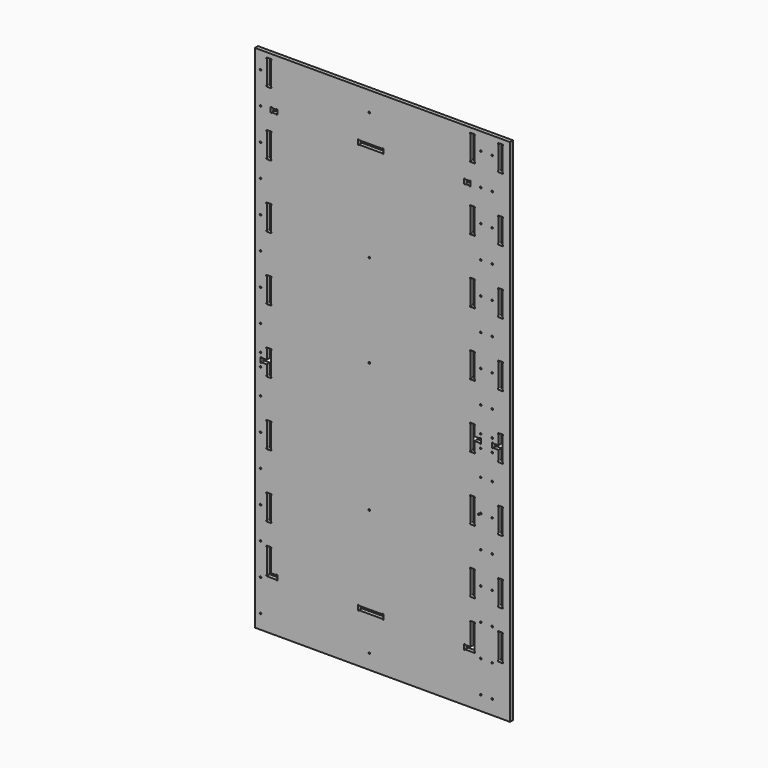
from build123d import *

# Parameters (mm, degrees)
F1_DEPTH = 18


# Not quite as in the source:
# - ends of sketch curves that miss each other by under 0.0002 mm in the source are joined


with BuildPart() as f1:
    # F0 (on Front) → F1 (new body)
    with BuildSketch(Plane.XZ):
        Polygon((-600, 1199.490696), (-600, -1200), (599.527337, -1200), (599.50121, 1199.503749), align=None)
        with BuildLine():
            ThreePointArc((-573.493655, -1128.773735), (-570.8420045706, -1129.8720845706), (-569.743655, -1132.523735))
            ThreePointArc((-569.743655, -1132.523735), (-570.8420045706, -1135.1753854294), (-573.493655, -1136.273735))
            ThreePointArc((-573.493655, -1136.273735), (-576.1453054294, -1135.1753854294), (-577.243655, -1132.523735))
            ThreePointArc((-577.243655, -1132.523735), (-576.1453054294, -1129.8720845706), (-573.493655, -1128.773735))
        make_face(mode=Mode.SUBTRACT)
        with BuildLine():
            ThreePointArc((-573.493655, -978.773735), (-570.8420045706, -979.8720845706), (-569.743655, -982.523735))
            ThreePointArc((-569.743655, -982.523735), (-570.8420045706, -985.1753854294), (-573.493655, -986.273735))
            ThreePointArc((-573.493655, -986.273735), (-576.1453054294, -985.1753854294), (-577.243655, -982.523735))
            ThreePointArc((-577.243655, -982.523735), (-576.1453054294, -979.8720845706), (-573.493655, -978.773735))
        make_face(mode=Mode.SUBTRACT)
        with BuildLine():
            ThreePointArc((-543.727655065, -848.5071848473), (-546.7362958526, -845.1312101747), (-543.477726, -841.9957920376))
            Line((-543.477726, -841.9957920376), (-524.977539, -841.99559))
            ThreePointArc((-524.977539, -841.99559), (-521.7198869029, -845.1309746571), (-524.7274680238, -848.5069766909))
            Line((-524.7274680238, -848.5069766909), (-524.726366, -949.761986))
            Line((-524.726366, -949.761986), (-500.237725, -949.76172))
            ThreePointArc((-500.237725, -949.76172), (-496.8617502129, -946.7530791459), (-493.7263320376, -950.011649))
            Line((-493.7263320376, -950.011649), (-493.726131, -968.511667))
            ThreePointArc((-493.726131, -968.511667), (-496.8615156571, -971.7693190971), (-500.2375176909, -968.7617379762))
            Line((-500.2375176909, -968.7617379762), (-543.476346, -968.762208))
            ThreePointArc((-543.476346, -968.762208), (-546.7339980971, -965.6268233429), (-543.7264169762, -962.2508213091))
            Line((-543.7264169762, -962.2508213091), (-543.727655065, -848.5071848473))
        make_face(mode=Mode.SUBTRACT)
        with BuildLine():
            ThreePointArc((-573.493655, -828.773735), (-570.8420045706, -829.8720845706), (-569.743655, -832.523735))
            ThreePointArc((-569.743655, -832.523735), (-570.8420045706, -835.1753854294), (-573.493655, -836.273735))
            ThreePointArc((-573.493655, -836.273735), (-576.1453054294, -835.1753854294), (-577.243655, -832.523735))
            ThreePointArc((-577.243655, -832.523735), (-576.1453054294, -829.8720845706), (-573.493655, -828.773735))
        make_face(mode=Mode.SUBTRACT)
        with BuildLine():
            ThreePointArc((-573.493655, -678.773735), (-570.8420045706, -679.8720845706), (-569.743655, -682.523735))
            ThreePointArc((-569.743655, -682.523735), (-570.8420045706, -685.1753854294), (-573.493655, -686.273735))
            ThreePointArc((-573.493655, -686.273735), (-576.1453054294, -685.1753854294), (-577.243655, -682.523735))
            ThreePointArc((-577.243655, -682.523735), (-576.1453054294, -679.8720845706), (-573.493655, -678.773735))
        make_face(mode=Mode.SUBTRACT)
        with BuildLine():
            ThreePointArc((-524.980091, -621.9929560323), (-521.7224389029, -625.1283406571), (-524.7300200238, -628.5043426909))
            Line((-524.7300200238, -628.5043426909), (-524.728845, -736.481683))
            ThreePointArc((-524.728845, -736.481683), (-521.7202041651, -739.8576582867), (-524.978775, -742.9930759623))
            Line((-524.978775, -742.9930759623), (-543.478594, -742.993277))
            ThreePointArc((-543.478594, -742.993277), (-546.7362460971, -739.8578923429), (-543.7286649762, -736.4818903091))
            Line((-543.7286649762, -736.4818903091), (-543.72984, -628.50455))
            ThreePointArc((-543.72984, -628.50455), (-546.7384808541, -625.1285752129), (-543.479911, -621.9931570376))
            Line((-543.479911, -621.9931570376), (-524.980091, -621.9929560323))
        make_face(mode=Mode.SUBTRACT)
        with BuildLine():
            ThreePointArc((-65.644873, -1130.966953), (-64.5465234294, -1128.3153025706), (-61.894873, -1127.216953))
            ThreePointArc((-61.894873, -1127.216953), (-59.2432225706, -1128.3153025706), (-58.144873, -1130.966953))
            ThreePointArc((-58.144873, -1130.966953), (-59.2432225706, -1133.6186034294), (-61.894873, -1134.716953))
            ThreePointArc((-61.894873, -1134.716953), (-64.5465234294, -1133.6186034294), (-65.644873, -1130.966953))
        make_face(mode=Mode.SUBTRACT)
        with BuildLine():
            ThreePointArc((-116.2255609677, -950.007539), (-113.0901763429, -946.7498869029), (-109.7141743091, -949.7574680238))
            Line((-109.7141743091, -949.7574680238), (-1.737032, -949.756293))
            ThreePointArc((-1.737032, -949.756293), (1.6389427871, -946.7476521459), (4.7743609624, -950.006222))
            Line((4.7743609624, -950.006222), (4.774562, -968.50624))
            ThreePointArc((4.774562, -968.50624), (1.6391773429, -971.7638920971), (-1.7368246909, -968.7563109762))
            Line((-1.7368246909, -968.7563109762), (-109.713967, -968.757486))
            ThreePointArc((-109.713967, -968.757486), (-113.0899408253, -971.7661268526), (-116.2253589624, -968.507557))
            Line((-116.2253589624, -968.507557), (-116.2255609677, -950.007539))
        make_face(mode=Mode.SUBTRACT)
        with BuildLine():
            ThreePointArc((-573.493655, -528.773735), (-570.8420045706, -529.8720845706), (-569.743655, -532.523735))
            ThreePointArc((-569.743655, -532.523735), (-570.8420045706, -535.1753854294), (-573.493655, -536.273735))
            ThreePointArc((-573.493655, -536.273735), (-576.1453054294, -535.1753854294), (-577.243655, -532.523735))
            ThreePointArc((-577.243655, -532.523735), (-576.1453054294, -529.8720845706), (-573.493655, -528.773735))
        make_face(mode=Mode.SUBTRACT)
        with BuildLine():
            ThreePointArc((-573.493655, -378.773735), (-570.8420045706, -379.8720845706), (-569.743655, -382.523735))
            ThreePointArc((-569.743655, -382.523735), (-570.8420045706, -385.1753854294), (-573.493655, -386.273735))
            ThreePointArc((-573.493655, -386.273735), (-576.1453054294, -385.1753854294), (-577.243655, -382.523735))
            ThreePointArc((-577.243655, -382.523735), (-576.1453054294, -379.8720845706), (-573.493655, -378.773735))
        make_face(mode=Mode.SUBTRACT)
        with BuildLine():
            ThreePointArc((-524.983356, -321.9926560323), (-521.7257039029, -325.1280406571), (-524.7332850238, -328.5040426909))
            Line((-524.7332850238, -328.5040426909), (-524.73211, -436.481383))
            ThreePointArc((-524.73211, -436.481383), (-521.7234691459, -439.8573577871), (-524.982039, -442.9927759624))
            Line((-524.982039, -442.9927759624), (-543.481858, -442.992977))
            ThreePointArc((-543.481858, -442.992977), (-546.7395100971, -439.8575923429), (-543.7319289762, -436.4815903091))
            Line((-543.7319289762, -436.4815903091), (-543.733104, -328.50425))
            ThreePointArc((-543.733104, -328.50425), (-546.7417448541, -325.1282752129), (-543.483175, -321.9928570376))
            Line((-543.483175, -321.9928570376), (-524.983356, -321.9926560323))
        make_face(mode=Mode.SUBTRACT)
        with BuildLine():
            ThreePointArc((-573.493655, -228.773735), (-570.8420045706, -229.8720845706), (-569.743655, -232.523735))
            ThreePointArc((-569.743655, -232.523735), (-570.8420045706, -235.1753854294), (-573.493655, -236.273735))
            ThreePointArc((-573.493655, -236.273735), (-576.1453054294, -235.1753854294), (-577.243655, -232.523735))
            ThreePointArc((-577.243655, -232.523735), (-576.1453054294, -229.8720845706), (-573.493655, -228.773735))
        make_face(mode=Mode.SUBTRACT)
        with BuildLine():
            ThreePointArc((-573.493655, -108.773735), (-570.8420045706, -109.8720845706), (-569.743655, -112.523735))
            ThreePointArc((-569.743655, -112.523735), (-570.8420045706, -115.1753854294), (-573.493655, -116.273735))
            ThreePointArc((-573.493655, -116.273735), (-576.1453054294, -115.1753854294), (-577.243655, -112.523735))
            ThreePointArc((-577.243655, -112.523735), (-576.1453054294, -109.8720845706), (-573.493655, -108.773735))
        make_face(mode=Mode.SUBTRACT)
        with BuildLine():
            ThreePointArc((-524.98662, -21.9923560324), (-521.7289688837, -25.1277411567), (-524.7365500238, -28.5037426909))
            Line((-524.7365500238, -28.5037426909), (-524.735375, -136.481083))
            ThreePointArc((-524.735375, -136.481083), (-521.7267341459, -139.8570577871), (-524.985304, -142.9924759624))
            Line((-524.985304, -142.9924759624), (-543.485097, -142.992677))
            ThreePointArc((-543.485097, -142.992677), (-546.7429566344, -139.8575125023), (-543.7356079554, -136.4813075779))
            Line((-543.7356079554, -136.4813075779), (-543.73916, -91.996839))
            Line((-543.73916, -91.996839), (-568.227835, -91.997105))
            ThreePointArc((-568.227835, -91.997105), (-571.6038097871, -95.0057458541), (-574.7392279624, -91.747176))
            Line((-574.7392279624, -91.747176), (-574.739429, -73.247158))
            ThreePointArc((-574.739429, -73.247158), (-571.6040443429, -69.9895059029), (-568.2280423091, -72.9970870238))
            Line((-568.2280423091, -72.9970870238), (-543.739563, -72.996821))
            Line((-543.739563, -72.996821), (-543.736807, -28.503931))
            ThreePointArc((-543.736807, -28.503931), (-546.7452018944, -25.1277420055), (-543.486412, -21.9925570804))
            Line((-543.486412, -21.9925570804), (-524.98662, -21.9923560324))
        make_face(mode=Mode.SUBTRACT)
        with BuildLine():
            ThreePointArc((-573.493655, -48.773735), (-570.8420045706, -49.8720845706), (-569.743655, -52.523735))
            ThreePointArc((-569.743655, -52.523735), (-570.8420045706, -55.1753854294), (-573.493655, -56.273735))
            ThreePointArc((-573.493655, -56.273735), (-576.1453054294, -55.1753854294), (-577.243655, -52.523735))
            ThreePointArc((-577.243655, -52.523735), (-576.1453054294, -49.8720845706), (-573.493655, -48.773735))
        make_face(mode=Mode.SUBTRACT)
        with BuildLine():
            ThreePointArc((-65.644873, -537.813487), (-64.5465234294, -535.1618365706), (-61.894873, -534.063487))
            ThreePointArc((-61.894873, -534.063487), (-59.2432225706, -535.1618365706), (-58.144873, -537.813487))
            ThreePointArc((-58.144873, -537.813487), (-59.2432225706, -540.4651374294), (-61.894873, -541.563487))
            ThreePointArc((-61.894873, -541.563487), (-64.5465234294, -540.4651374294), (-65.644873, -537.813487))
        make_face(mode=Mode.SUBTRACT)
        with BuildLine():
            ThreePointArc((413.2732930585, -848.4955412375), (410.2646479537, -845.1195722402), (413.523212, -841.9841500368))
            Line((413.523212, -841.9841500368), (432.023061, -841.983948))
            ThreePointArc((432.023061, -841.983948), (435.2807130971, -845.1193326571), (432.2731319762, -848.4953346909))
            Line((432.2731319762, -848.4953346909), (432.27437, -962.240198))
            ThreePointArc((432.27437, -962.240198), (435.2830108541, -965.6161727871), (432.024441, -968.7515909624))
            Line((432.024441, -968.7515909624), (388.786108, -968.752061))
            ThreePointArc((388.786108, -968.752061), (385.4101332129, -971.7607018541), (382.2747150376, -968.502132))
            Line((382.2747150376, -968.502132), (382.274514, -950.002325))
            ThreePointArc((382.274514, -950.002325), (385.4098986571, -946.7446729029), (388.7859006909, -949.7522540238))
            Line((388.7859006909, -949.7522540238), (413.274542, -949.751987))
            Line((413.274542, -949.751987), (413.2732930585, -848.4955412375))
        make_face(mode=Mode.SUBTRACT)
        with BuildLine():
            ThreePointArc((461.992992, -1128.773735), (464.6446424294, -1129.8720845706), (465.742992, -1132.523735))
            ThreePointArc((465.742992, -1132.523735), (464.6446424294, -1135.1753854294), (461.992992, -1136.273735))
            ThreePointArc((461.992992, -1136.273735), (459.3413415706, -1135.1753854294), (458.242992, -1132.523735))
            ThreePointArc((458.242992, -1132.523735), (459.3413415706, -1129.8720845706), (461.992992, -1128.773735))
        make_face(mode=Mode.SUBTRACT)
        with BuildLine():
            ThreePointArc((515.501657, -1128.773735), (518.1533074294, -1129.8720845706), (519.251657, -1132.523735))
            ThreePointArc((519.251657, -1132.523735), (518.1533074294, -1135.1753854294), (515.501657, -1136.273735))
            ThreePointArc((515.501657, -1136.273735), (512.8500065706, -1135.1753854294), (511.751657, -1132.523735))
            ThreePointArc((511.751657, -1132.523735), (512.8500065706, -1129.8720845706), (515.501657, -1128.773735))
        make_face(mode=Mode.SUBTRACT)
        with BuildLine():
            ThreePointArc((461.992992, -978.773735), (464.6446424294, -979.8720845706), (465.742992, -982.523735))
            ThreePointArc((465.742992, -982.523735), (464.6446424294, -985.1753854294), (461.992992, -986.273735))
            ThreePointArc((461.992992, -986.273735), (459.3413415706, -985.1753854294), (458.242992, -982.523735))
            ThreePointArc((458.242992, -982.523735), (459.3413415706, -979.8720845706), (461.992992, -978.773735))
        make_face(mode=Mode.SUBTRACT)
        with BuildLine():
            ThreePointArc((515.501657, -978.773735), (518.1533074294, -979.8720845706), (519.251657, -982.523735))
            ThreePointArc((519.251657, -982.523735), (518.1533074294, -985.1753854294), (515.501657, -986.273735))
            ThreePointArc((515.501657, -986.273735), (512.8500065706, -985.1753854294), (511.751657, -982.523735))
            ThreePointArc((511.751657, -982.523735), (512.8500065706, -979.8720845706), (515.501657, -978.773735))
        make_face(mode=Mode.SUBTRACT)
        with BuildLine():
            Line((545.274457, -962.243698), (545.273219, -848.49533))
            ThreePointArc((545.273219, -848.49533), (542.2645781474, -845.1193561747), (545.523148, -841.9839380376))
            Line((545.523148, -841.9839380376), (564.022958, -841.983736))
            ThreePointArc((564.022958, -841.983736), (567.2806100971, -845.1191206571), (564.2730289762, -848.4951226909))
            Line((564.2730289762, -848.4951226909), (564.274266, -962.243491))
            ThreePointArc((564.274266, -962.243491), (567.2829068541, -965.6194657871), (564.024337, -968.7548839624))
            Line((564.024337, -968.7548839624), (545.524528, -968.755085))
            ThreePointArc((545.524528, -968.755085), (542.2668759029, -965.6197003429), (545.274457, -962.243698))
        make_face(mode=Mode.SUBTRACT)
        with BuildLine():
            ThreePointArc((413.522136, -742.9794189677), (410.2644839029, -739.8440343429), (413.2720650238, -736.4680323091))
            Line((413.2720650238, -736.4680323091), (413.27089, -628.49064))
            ThreePointArc((413.27089, -628.49064), (410.2622491459, -625.1146652129), (413.520819, -621.9792470376))
            Line((413.520819, -621.9792470376), (432.020837, -621.979046))
            ThreePointArc((432.020837, -621.979046), (435.2784890971, -625.1144306571), (432.2709079762, -628.4904326909))
            Line((432.2709079762, -628.4904326909), (432.272083, -736.467825))
            ThreePointArc((432.272083, -736.467825), (435.2807238526, -739.8437988253), (432.022154, -742.9792169624))
            Line((432.022154, -742.9792169624), (413.522136, -742.9794189677))
        make_face(mode=Mode.SUBTRACT)
        with BuildLine():
            ThreePointArc((461.992992, -828.773735), (464.6446424294, -829.8720845706), (465.742992, -832.523735))
            ThreePointArc((465.742992, -832.523735), (464.6446424294, -835.1753854294), (461.992992, -836.273735))
            ThreePointArc((461.992992, -836.273735), (459.3413415706, -835.1753854294), (458.242992, -832.523735))
            ThreePointArc((458.242992, -832.523735), (459.3413415706, -829.8720845706), (461.992992, -828.773735))
        make_face(mode=Mode.SUBTRACT)
        with BuildLine():
            ThreePointArc((515.501657, -828.773735), (518.1533074294, -829.8720845706), (519.251657, -832.523735))
            ThreePointArc((519.251657, -832.523735), (518.1533074294, -835.1753854294), (515.501657, -836.273735))
            ThreePointArc((515.501657, -836.273735), (512.8500065706, -835.1753854294), (511.751657, -832.523735))
            ThreePointArc((511.751657, -832.523735), (512.8500065706, -829.8720845706), (515.501657, -828.773735))
        make_face(mode=Mode.SUBTRACT)
        with BuildLine():
            ThreePointArc((461.992992, -678.773735), (464.6446424294, -679.8720845706), (465.742992, -682.523735))
            ThreePointArc((465.742992, -682.523735), (464.6446424294, -685.1753854294), (461.992992, -686.273735))
            ThreePointArc((461.992992, -686.273735), (459.3413415706, -685.1753854294), (458.242992, -682.523735))
            ThreePointArc((458.242992, -682.523735), (459.3413415706, -679.8720845706), (461.992992, -678.773735))
        make_face(mode=Mode.SUBTRACT)
        with BuildLine():
            ThreePointArc((515.501657, -678.773735), (518.1533074294, -679.8720845706), (519.251657, -682.523735))
            ThreePointArc((519.251657, -682.523735), (518.1533074294, -685.1753854294), (515.501657, -686.273735))
            ThreePointArc((515.501657, -686.273735), (512.8500065706, -685.1753854294), (511.751657, -682.523735))
            ThreePointArc((511.751657, -682.523735), (512.8500065706, -679.8720845706), (515.501657, -678.773735))
        make_face(mode=Mode.SUBTRACT)
        with BuildLine():
            ThreePointArc((545.522316, -742.9779789677), (542.2646629037, -739.8425933813), (545.272244947, -736.4665903121))
            Line((545.272244947, -736.4665903121), (545.27107, -628.489199))
            ThreePointArc((545.27107, -628.489199), (542.2624291459, -625.1132242129), (545.520999, -621.9778060376))
            Line((545.520999, -621.9778060376), (564.020799, -621.977605))
            ThreePointArc((564.020799, -621.977605), (567.2784510971, -625.1129896571), (564.2708699762, -628.4889916909))
            Line((564.2708699762, -628.4889916909), (564.272045, -736.466332))
            ThreePointArc((564.272045, -736.466332), (567.2806858526, -739.8423058253), (564.022116, -742.9777239624))
            Line((564.022116, -742.9777239624), (545.522316, -742.9779789677))
        make_face(mode=Mode.SUBTRACT)
        with BuildLine():
            ThreePointArc((432.268818065, -436.4675241527), (435.2774588526, -439.8434988253), (432.018889, -442.9789169624))
            Line((432.018889, -442.9789169624), (413.518871, -442.979119))
            ThreePointArc((413.518871, -442.979119), (410.2612189029, -439.8437343429), (413.2688000238, -436.4677323091))
            Line((413.2688000238, -436.4677323091), (413.267625, -328.49034))
            ThreePointArc((413.267625, -328.49034), (410.2589841459, -325.1143652129), (413.517554, -321.9789470376))
            Line((413.517554, -321.9789470376), (432.017572, -321.978746))
            ThreePointArc((432.017572, -321.978746), (435.2752240971, -325.1141306571), (432.2676429762, -328.4901326909))
            Line((432.2676429762, -328.4901326909), (432.268818065, -436.4675241527))
        make_face(mode=Mode.SUBTRACT)
        with BuildLine():
            ThreePointArc((461.992992, -528.773735), (464.6446424294, -529.8720845706), (465.742992, -532.523735))
            ThreePointArc((465.742992, -532.523735), (464.6446424294, -535.1753854294), (461.992992, -536.273735))
            ThreePointArc((461.992992, -536.273735), (459.3413415706, -535.1753854294), (458.242992, -532.523735))
            ThreePointArc((458.242992, -532.523735), (459.3413415706, -529.8720845706), (461.992992, -528.773735))
        make_face(mode=Mode.SUBTRACT)
        with BuildLine():
            ThreePointArc((515.501657, -528.773735), (518.1533074294, -529.8720845706), (519.251657, -532.523735))
            ThreePointArc((519.251657, -532.523735), (518.1533074294, -535.1753854294), (515.501657, -536.273735))
            ThreePointArc((515.501657, -536.273735), (512.8500065706, -535.1753854294), (511.751657, -532.523735))
            ThreePointArc((511.751657, -532.523735), (512.8500065706, -529.8720845706), (515.501657, -528.773735))
        make_face(mode=Mode.SUBTRACT)
        with BuildLine():
            ThreePointArc((447.984, -388.548053), (449.0823495706, -385.8964025706), (451.734, -384.798053))
            ThreePointArc((451.734, -384.798053), (454.3856504294, -385.8964025706), (455.484, -388.548053))
            ThreePointArc((455.484, -388.548053), (454.3856504294, -391.1997034294), (451.734, -392.298053))
            ThreePointArc((451.734, -392.298053), (449.0823495706, -391.1997034294), (447.984, -388.548053))
        make_face(mode=Mode.SUBTRACT)
        with BuildLine():
            ThreePointArc((461.992992, -378.773735), (464.6446424294, -379.8720845706), (465.742992, -382.523735))
            ThreePointArc((465.742992, -382.523735), (464.6446424294, -385.1753854294), (461.992992, -386.273735))
            ThreePointArc((461.992992, -386.273735), (459.3413415706, -385.1753854294), (458.242992, -382.523735))
            ThreePointArc((458.242992, -382.523735), (459.3413415706, -379.8720845706), (461.992992, -378.773735))
        make_face(mode=Mode.SUBTRACT)
        with BuildLine():
            ThreePointArc((515.501657, -378.773735), (518.1533074294, -379.8720845706), (519.251657, -382.523735))
            ThreePointArc((519.251657, -382.523735), (518.1533074294, -385.1753854294), (515.501657, -386.273735))
            ThreePointArc((515.501657, -386.273735), (512.8500065706, -385.1753854294), (511.751657, -382.523735))
            ThreePointArc((511.751657, -382.523735), (512.8500065706, -379.8720845706), (515.501657, -378.773735))
        make_face(mode=Mode.SUBTRACT)
        with BuildLine():
            ThreePointArc((545.519052, -442.9776789677), (542.2613989228, -439.8422938795), (545.2689799529, -436.4662903887))
            Line((545.2689799529, -436.4662903887), (545.267805, -328.488899))
            ThreePointArc((545.267805, -328.488899), (542.2591641651, -325.1129237133), (545.517735, -321.9775060377))
            Line((545.517735, -321.9775060377), (564.017534, -321.977305))
            ThreePointArc((564.017534, -321.977305), (567.2751860971, -325.1126896571), (564.2676049762, -328.4886916909))
            Line((564.2676049762, -328.4886916909), (564.26878, -436.466032))
            ThreePointArc((564.26878, -436.466032), (567.2774208526, -439.8420058253), (564.018851, -442.9774239624))
            Line((564.018851, -442.9774239624), (545.519052, -442.9776789677))
        make_face(mode=Mode.SUBTRACT)
        with BuildLine():
            ThreePointArc((432.2652829744, -136.4718953334), (435.2740837852, -139.8477271674), (432.015663, -142.9832999823))
            Line((432.015663, -142.9832999823), (413.515627, -142.983501))
            ThreePointArc((413.515627, -142.983501), (410.2579749029, -139.8481163429), (413.2655560238, -136.4721143091))
            Line((413.2655560238, -136.4721143091), (413.264381, -28.494722))
            ThreePointArc((413.264381, -28.494722), (410.2557401666, -25.1187476751), (413.514311, -21.9833300377))
            Line((413.514311, -21.9833300377), (432.014348, -21.983128))
            ThreePointArc((432.014348, -21.983128), (435.2718385306, -25.1186802863), (432.2640839659, -28.4945275573))
            Line((432.2640839659, -28.4945275573), (432.262235, -72.9862))
            Line((432.262235, -72.9862), (456.75085, -72.985934))
            ThreePointArc((456.75085, -72.985934), (460.1268238253, -69.9772931474), (463.2622419624, -73.235863))
            Line((463.2622419624, -73.235863), (463.262444, -91.735881))
            ThreePointArc((463.262444, -91.735881), (460.1270593429, -94.9935330971), (456.7510573091, -91.9859519762))
            Line((456.7510573091, -91.9859519762), (432.262638, -91.986218))
            Line((432.262638, -91.986218), (432.2652829744, -136.4718953334))
        make_face(mode=Mode.SUBTRACT)
        with BuildLine():
            ThreePointArc((461.992992, -228.773735), (464.6446424294, -229.8720845706), (465.742992, -232.523735))
            ThreePointArc((465.742992, -232.523735), (464.6446424294, -235.1753854294), (461.992992, -236.273735))
            ThreePointArc((461.992992, -236.273735), (459.3413415706, -235.1753854294), (458.242992, -232.523735))
            ThreePointArc((458.242992, -232.523735), (459.3413415706, -229.8720845706), (461.992992, -228.773735))
        make_face(mode=Mode.SUBTRACT)
        with BuildLine():
            ThreePointArc((515.501657, -228.773735), (518.1533074294, -229.8720845706), (519.251657, -232.523735))
            ThreePointArc((519.251657, -232.523735), (518.1533074294, -235.1753854294), (515.501657, -236.273735))
            ThreePointArc((515.501657, -236.273735), (512.8500065706, -235.1753854294), (511.751657, -232.523735))
            ThreePointArc((511.751657, -232.523735), (512.8500065706, -229.8720845706), (515.501657, -228.773735))
        make_face(mode=Mode.SUBTRACT)
        with BuildLine():
            ThreePointArc((461.992992, -108.773735), (464.6446424294, -109.8720845706), (465.742992, -112.523735))
            ThreePointArc((465.742992, -112.523735), (464.6446424294, -115.1753854294), (461.992992, -116.273735))
            ThreePointArc((461.992992, -116.273735), (459.3413415706, -115.1753854294), (458.242992, -112.523735))
            ThreePointArc((458.242992, -112.523735), (459.3413415706, -109.8720845706), (461.992992, -108.773735))
        make_face(mode=Mode.SUBTRACT)
        with BuildLine():
            ThreePointArc((515.501657, -108.773735), (518.1533074294, -109.8720845706), (519.251657, -112.523735))
            ThreePointArc((519.251657, -112.523735), (518.1533074294, -115.1753854294), (515.501657, -116.273735))
            ThreePointArc((515.501657, -116.273735), (512.8500065706, -115.1753854294), (511.751657, -112.523735))
            ThreePointArc((511.751657, -112.523735), (512.8500065706, -109.8720845706), (515.501657, -108.773735))
        make_face(mode=Mode.SUBTRACT)
        with BuildLine():
            ThreePointArc((461.992992, -48.773735), (464.6446424294, -49.8720845706), (465.742992, -52.523735))
            ThreePointArc((465.742992, -52.523735), (464.6446424294, -55.1753854294), (461.992992, -56.273735))
            ThreePointArc((461.992992, -56.273735), (459.3413415706, -55.1753854294), (458.242992, -52.523735))
            ThreePointArc((458.242992, -52.523735), (459.3413415706, -49.8720845706), (461.992992, -48.773735))
        make_face(mode=Mode.SUBTRACT)
        with BuildLine():
            ThreePointArc((515.501657, -48.773735), (518.1533074294, -49.8720845706), (519.251657, -52.523735))
            ThreePointArc((519.251657, -52.523735), (518.1533074294, -55.1753854294), (515.501657, -56.273735))
            ThreePointArc((515.501657, -56.273735), (512.8500065706, -55.1753854294), (511.751657, -52.523735))
            ThreePointArc((511.751657, -52.523735), (512.8500065706, -49.8720845706), (515.501657, -48.773735))
        make_face(mode=Mode.SUBTRACT)
        with BuildLine():
            ThreePointArc((545.513838, -142.9839189899), (542.2559918459, -139.8487409931), (545.2633540444, -136.4725485752))
            Line((545.2633540444, -136.4725485752), (545.25999, -91.98499))
            Line((545.25999, -91.98499), (520.771316, -91.985256))
            ThreePointArc((520.771316, -91.985256), (517.3953421747, -94.9938968526), (514.2599240376, -91.735327))
            Line((514.2599240376, -91.735327), (514.259723, -73.235309))
            ThreePointArc((514.259723, -73.235309), (517.3951076571, -69.9776569029), (520.7711096909, -72.9852380238))
            Line((520.7711096909, -72.9852380238), (545.259783, -72.984972))
            Line((545.259783, -72.984972), (545.262179, -28.495176))
            ThreePointArc((545.262179, -28.495176), (542.2537571036, -25.1190100629), (545.512522, -21.9837990747))
            Line((545.512522, -21.9837990747), (564.012515, -21.983598))
            ThreePointArc((564.012515, -21.983598), (567.2701670971, -25.1189826571), (564.2625859762, -28.4949846909))
            Line((564.2625859762, -28.4949846909), (564.263761, -136.472325))
            ThreePointArc((564.263761, -136.472325), (567.2724018541, -139.8482997871), (564.013832, -142.9837179624))
            Line((564.013832, -142.9837179624), (545.513838, -142.9839189899))
        make_face(mode=Mode.SUBTRACT)
        with BuildLine():
            ThreePointArc((-573.493655, 71.226265), (-570.8420045706, 70.1279154294), (-569.743655, 67.476265))
            ThreePointArc((-569.743655, 67.476265), (-570.8420045706, 64.8246145706), (-573.493655, 63.726265))
            ThreePointArc((-573.493655, 63.726265), (-576.1453054294, 64.8246145706), (-577.243655, 67.476265))
            ThreePointArc((-577.243655, 67.476265), (-576.1453054294, 70.1279154294), (-573.493655, 71.226265))
        make_face(mode=Mode.SUBTRACT)
        with BuildLine():
            ThreePointArc((-573.493655, 221.226265), (-570.8420045706, 220.1279154294), (-569.743655, 217.476265))
            ThreePointArc((-569.743655, 217.476265), (-570.8420045706, 214.8246145706), (-573.493655, 213.726265))
            ThreePointArc((-573.493655, 213.726265), (-576.1453054294, 214.8246145706), (-577.243655, 217.476265))
            ThreePointArc((-577.243655, 217.476265), (-576.1453054294, 220.1279154294), (-573.493655, 221.226265))
        make_face(mode=Mode.SUBTRACT)
        with BuildLine():
            ThreePointArc((-543.7396339887, 271.4963501468), (-546.7482748349, 274.8723252867), (-543.489704, 278.0077429623))
            Line((-543.489704, 278.0077429623), (-524.989885, 278.007944))
            ThreePointArc((-524.989885, 278.007944), (-521.7322329029, 274.8725593429), (-524.7398140238, 271.4965573091))
            Line((-524.7398140238, 271.4965573091), (-524.738639, 163.519217))
            ThreePointArc((-524.738639, 163.519217), (-521.7299981459, 160.1432422129), (-524.988568, 157.0078240376))
            Line((-524.988568, 157.0078240376), (-543.488388, 157.007623))
            ThreePointArc((-543.488388, 157.007623), (-546.7460400971, 160.1430076571), (-543.7384589762, 163.5190096909))
            Line((-543.7384589762, 163.5190096909), (-543.7396339887, 271.4963501468))
        make_face(mode=Mode.SUBTRACT)
        with BuildLine():
            ThreePointArc((-573.493655, 371.226265), (-570.8420045706, 370.1279154294), (-569.743655, 367.476265))
            ThreePointArc((-569.743655, 367.476265), (-570.8420045706, 364.8246145706), (-573.493655, 363.726265))
            ThreePointArc((-573.493655, 363.726265), (-576.1453054294, 364.8246145706), (-577.243655, 367.476265))
            ThreePointArc((-577.243655, 367.476265), (-576.1453054294, 370.1279154294), (-573.493655, 371.226265))
        make_face(mode=Mode.SUBTRACT)
        with BuildLine():
            ThreePointArc((-573.493655, 521.226265), (-570.8420045706, 520.1279154294), (-569.743655, 517.476265))
            ThreePointArc((-569.743655, 517.476265), (-570.8420045706, 514.8246145706), (-573.493655, 513.726265))
            ThreePointArc((-573.493655, 513.726265), (-576.1453054294, 514.8246145706), (-577.243655, 517.476265))
            ThreePointArc((-577.243655, 517.476265), (-576.1453054294, 520.1279154294), (-573.493655, 521.226265))
        make_face(mode=Mode.SUBTRACT)
        with BuildLine():
            ThreePointArc((-524.99315, 578.0082439677), (-521.7354979029, 574.8728593429), (-524.7430790238, 571.4968573091))
            Line((-524.7430790238, 571.4968573091), (-524.741904, 463.519517))
            ThreePointArc((-524.741904, 463.519517), (-521.7332631459, 460.1435422129), (-524.991833, 457.0081240376))
            Line((-524.991833, 457.0081240376), (-543.491652, 457.007923))
            ThreePointArc((-543.491652, 457.007923), (-546.7493040971, 460.1433076571), (-543.7417229762, 463.5193096909))
            Line((-543.7417229762, 463.5193096909), (-543.742898, 571.49665))
            ThreePointArc((-543.742898, 571.49665), (-546.7515388541, 574.8726247871), (-543.492969, 578.0080429624))
            Line((-543.492969, 578.0080429624), (-524.99315, 578.0082439677))
        make_face(mode=Mode.SUBTRACT)
        with BuildLine():
            ThreePointArc((-65.644873, 70.75488), (-64.5465234294, 73.4065304294), (-61.894873, 74.50488))
            ThreePointArc((-61.894873, 74.50488), (-59.2432225706, 73.4065304294), (-58.144873, 70.75488))
            ThreePointArc((-58.144873, 70.75488), (-59.2432225706, 68.1032295706), (-61.894873, 67.00488))
            ThreePointArc((-61.894873, 67.00488), (-64.5465234294, 68.1032295706), (-65.644873, 70.75488))
        make_face(mode=Mode.SUBTRACT)
        with BuildLine():
            ThreePointArc((-65.644873, 506.390807), (-64.5465234294, 509.0424574294), (-61.894873, 510.140807))
            ThreePointArc((-61.894873, 510.140807), (-59.2432225706, 509.0424574294), (-58.144873, 506.390807))
            ThreePointArc((-58.144873, 506.390807), (-59.2432225706, 503.7391565706), (-61.894873, 502.640807))
            ThreePointArc((-61.894873, 502.640807), (-64.5465234294, 503.7391565706), (-65.644873, 506.390807))
        make_face(mode=Mode.SUBTRACT)
        with BuildLine():
            ThreePointArc((-573.493655, 671.226265), (-570.8420045706, 670.1279154294), (-569.743655, 667.476265))
            ThreePointArc((-569.743655, 667.476265), (-570.8420045706, 664.8246145706), (-573.493655, 663.726265))
            ThreePointArc((-573.493655, 663.726265), (-576.1453054294, 664.8246145706), (-577.243655, 667.476265))
            ThreePointArc((-577.243655, 667.476265), (-576.1453054294, 670.1279154294), (-573.493655, 671.226265))
        make_face(mode=Mode.SUBTRACT)
        with BuildLine():
            ThreePointArc((-573.493655, 821.226265), (-570.8420045706, 820.1279154294), (-569.743655, 817.476265))
            ThreePointArc((-569.743655, 817.476265), (-570.8420045706, 814.8246145706), (-573.493655, 813.726265))
            ThreePointArc((-573.493655, 813.726265), (-576.1453054294, 814.8246145706), (-577.243655, 817.476265))
            ThreePointArc((-577.243655, 817.476265), (-576.1453054294, 820.1279154294), (-573.493655, 821.226265))
        make_face(mode=Mode.SUBTRACT)
        with BuildLine():
            ThreePointArc((-543.7461629887, 871.4969501468), (-546.7548038541, 874.8729247871), (-543.496234, 878.0083429624))
            Line((-543.496234, 878.0083429624), (-524.996414, 878.008544))
            ThreePointArc((-524.996414, 878.008544), (-521.7387619029, 874.8731593429), (-524.7463430238, 871.4971573091))
            Line((-524.7463430238, 871.4971573091), (-524.745168, 763.519817))
            ThreePointArc((-524.745168, 763.519817), (-521.7365271459, 760.1438422129), (-524.995097, 757.0084240376))
            Line((-524.995097, 757.0084240376), (-543.494917, 757.008223))
            ThreePointArc((-543.494917, 757.008223), (-546.7525690971, 760.1436076571), (-543.7449879762, 763.5196096909))
            Line((-543.7449879762, 763.5196096909), (-543.7461629887, 871.4969501468))
        make_face(mode=Mode.SUBTRACT)
        with BuildLine():
            ThreePointArc((-573.493655, 971.226265), (-570.8420045706, 970.1279154294), (-569.743655, 967.476265))
            ThreePointArc((-569.743655, 967.476265), (-570.8420045706, 964.8246145706), (-573.493655, 963.726265))
            ThreePointArc((-573.493655, 963.726265), (-576.1453054294, 964.8246145706), (-577.243655, 967.476265))
            ThreePointArc((-577.243655, 967.476265), (-576.1453054294, 970.1279154294), (-573.493655, 971.226265))
        make_face(mode=Mode.SUBTRACT)
        with BuildLine():
            ThreePointArc((-501.2587058532, 977.0089919887), (-497.8827312129, 980.0176328541), (-494.7473130376, 976.759063))
            Line((-494.7473130376, 976.759063), (-494.747099, 958.258901))
            ThreePointArc((-494.747099, 958.258901), (-497.8824836571, 955.0012489029), (-501.2584856909, 958.0088300238))
            Line((-501.2584856909, 958.0088300238), (-519.235546, 958.008635))
            ThreePointArc((-519.235546, 958.008635), (-522.6115193257, 954.9999941282), (-525.7469379626, 958.258563))
            Line((-525.7469379626, 958.258563), (-525.747346, 976.758724))
            ThreePointArc((-525.747346, 976.758724), (-522.6119618411, 980.016376078), (-519.2359593857, 977.0087959703))
            Line((-519.2359593857, 977.0087959703), (-501.2587058532, 977.0089919887))
        make_face(mode=Mode.SUBTRACT)
        with BuildLine():
            ThreePointArc((-573.493655, 1121.226265), (-570.8420045706, 1120.1279154294), (-569.743655, 1117.476265))
            ThreePointArc((-569.743655, 1117.476265), (-570.8420045706, 1114.8246145706), (-573.493655, 1113.726265))
            ThreePointArc((-573.493655, 1113.726265), (-576.1453054294, 1114.8246145706), (-577.243655, 1117.476265))
            ThreePointArc((-577.243655, 1117.476265), (-576.1453054294, 1120.1279154294), (-573.493655, 1121.226265))
        make_face(mode=Mode.SUBTRACT)
        with BuildLine():
            ThreePointArc((-524.7484460113, 1063.5201168532), (-521.7398051459, 1060.1441422129), (-524.998375, 1057.0087240376))
            Line((-524.998375, 1057.0087240376), (-543.498393, 1057.008523))
            ThreePointArc((-543.498393, 1057.008523), (-546.7560450971, 1060.1439076571), (-543.7484639762, 1063.5199096909))
            Line((-543.7484639762, 1063.5199096909), (-543.749639, 1171.49725))
            ThreePointArc((-543.749639, 1171.49725), (-546.7582798541, 1174.8732247871), (-543.49971, 1178.0086429624))
            Line((-543.49971, 1178.0086429624), (-524.999692, 1178.008844))
            ThreePointArc((-524.999692, 1178.008844), (-521.7420399029, 1174.8734593429), (-524.7496210238, 1171.4974573091))
            Line((-524.7496210238, 1171.4974573091), (-524.7484460113, 1063.5201168532))
        make_face(mode=Mode.SUBTRACT)
        with BuildLine():
            ThreePointArc((-1.7581598473, 977.014427065), (1.6178143257, 980.0230678718), (4.7532329626, 976.764499))
            Line((4.7532329626, 976.764499), (4.753631, 958.264321))
            ThreePointArc((4.753631, 958.264321), (1.6182468411, 955.006668922), (-1.7577556143, 958.0142490297))
            Line((-1.7577556143, 958.0142490297), (-109.734896, 958.013074))
            ThreePointArc((-109.734896, 958.013074), (-113.1108697878, 955.0044331076), (-116.2462889627, 958.263001))
            Line((-116.2462889627, 958.263001), (-116.24689, 976.763179))
            ThreePointArc((-116.24689, 976.763179), (-113.1115063407, 980.0208320588), (-109.7355033857, 977.0132519703))
            Line((-109.7355033857, 977.0132519703), (-1.7581598473, 977.014427065))
        make_face(mode=Mode.SUBTRACT)
        with BuildLine():
            ThreePointArc((-65.644873, 1107.267947), (-64.5465234294, 1109.9195974294), (-61.894873, 1111.017947))
            ThreePointArc((-61.894873, 1111.017947), (-59.2432225706, 1109.9195974294), (-58.144873, 1107.267947))
            ThreePointArc((-58.144873, 1107.267947), (-59.2432225706, 1104.6162965706), (-61.894873, 1103.517947))
            ThreePointArc((-61.894873, 1103.517947), (-64.5465234294, 1104.6162965706), (-65.644873, 1107.267947))
        make_face(mode=Mode.SUBTRACT)
        with BuildLine():
            ThreePointArc((432.262289065, 163.5330758473), (435.2709298526, 160.1571011747), (432.01236, 157.0216830376))
            Line((432.01236, 157.0216830376), (413.512342, 157.021481))
            ThreePointArc((413.512342, 157.021481), (410.2546899029, 160.1568656571), (413.2622710238, 163.5328676909))
            Line((413.2622710238, 163.5328676909), (413.261096, 271.51026))
            ThreePointArc((413.261096, 271.51026), (410.2524551459, 274.8862347871), (413.511025, 278.0216529624))
            Line((413.511025, 278.0216529624), (432.011043, 278.021854))
            ThreePointArc((432.011043, 278.021854), (435.2686950971, 274.8864693429), (432.2611139762, 271.5104673091))
            Line((432.2611139762, 271.5104673091), (432.262289065, 163.5330758473))
        make_face(mode=Mode.SUBTRACT)
        with BuildLine():
            ThreePointArc((461.992992, 71.226265), (464.6446424294, 70.1279154294), (465.742992, 67.476265))
            ThreePointArc((465.742992, 67.476265), (464.6446424294, 64.8246145706), (461.992992, 63.726265))
            ThreePointArc((461.992992, 63.726265), (459.3413415706, 64.8246145706), (458.242992, 67.476265))
            ThreePointArc((458.242992, 67.476265), (459.3413415706, 70.1279154294), (461.992992, 71.226265))
        make_face(mode=Mode.SUBTRACT)
        with BuildLine():
            ThreePointArc((515.501657, 71.226265), (518.1533074294, 70.1279154294), (519.251657, 67.476265))
            ThreePointArc((519.251657, 67.476265), (518.1533074294, 64.8246145706), (515.501657, 63.726265))
            ThreePointArc((515.501657, 63.726265), (512.8500065706, 64.8246145706), (511.751657, 67.476265))
            ThreePointArc((511.751657, 67.476265), (512.8500065706, 70.1279154294), (515.501657, 71.226265))
        make_face(mode=Mode.SUBTRACT)
        with BuildLine():
            ThreePointArc((461.992992, 221.226265), (464.6446424294, 220.1279154294), (465.742992, 217.476265))
            ThreePointArc((465.742992, 217.476265), (464.6446424294, 214.8246145706), (461.992992, 213.726265))
            ThreePointArc((461.992992, 213.726265), (459.3413415706, 214.8246145706), (458.242992, 217.476265))
            ThreePointArc((458.242992, 217.476265), (459.3413415706, 220.1279154294), (461.992992, 221.226265))
        make_face(mode=Mode.SUBTRACT)
        with BuildLine():
            ThreePointArc((515.501657, 221.226265), (518.1533074294, 220.1279154294), (519.251657, 217.476265))
            ThreePointArc((519.251657, 217.476265), (518.1533074294, 214.8246145706), (515.501657, 213.726265))
            ThreePointArc((515.501657, 213.726265), (512.8500065706, 214.8246145706), (511.751657, 217.476265))
            ThreePointArc((511.751657, 217.476265), (512.8500065706, 220.1279154294), (515.501657, 221.226265))
        make_face(mode=Mode.SUBTRACT)
        with BuildLine():
            ThreePointArc((545.512523, 157.0229210323), (542.254870922, 160.1583051589), (545.2624510297, 163.5343076143))
            Line((545.2624510297, 163.5343076143), (545.261276, 271.511701))
            ThreePointArc((545.261276, 271.511701), (542.2526351459, 274.8876757871), (545.511205, 278.0230939624))
            Line((545.511205, 278.0230939624), (564.011005, 278.023295))
            ThreePointArc((564.011005, 278.023295), (567.2686570971, 274.8879103429), (564.2610759762, 271.5119083091))
            Line((564.2610759762, 271.5119083091), (564.262251, 163.534568))
            ThreePointArc((564.262251, 163.534568), (567.2708918526, 160.1585941747), (564.012322, 157.0231760376))
            Line((564.012322, 157.0231760376), (545.512523, 157.0229210323))
        make_face(mode=Mode.SUBTRACT)
        with BuildLine():
            ThreePointArc((432.259024065, 463.5333758473), (435.2676648526, 460.1574011747), (432.009095, 457.0219830376))
            Line((432.009095, 457.0219830376), (413.509077, 457.021781))
            ThreePointArc((413.509077, 457.021781), (410.2514249029, 460.1571656571), (413.2590060238, 463.5331676909))
            Line((413.2590060238, 463.5331676909), (413.257831, 571.51056))
            ThreePointArc((413.257831, 571.51056), (410.2491901459, 574.8865347871), (413.50776, 578.0219529624))
            Line((413.50776, 578.0219529624), (432.007778, 578.022154))
            ThreePointArc((432.007778, 578.022154), (435.2654300971, 574.8867693429), (432.2578489762, 571.5107673091))
            Line((432.2578489762, 571.5107673091), (432.259024065, 463.5333758473))
        make_face(mode=Mode.SUBTRACT)
        with BuildLine():
            ThreePointArc((461.992992, 371.226265), (464.6446424294, 370.1279154294), (465.742992, 367.476265))
            ThreePointArc((465.742992, 367.476265), (464.6446424294, 364.8246145706), (461.992992, 363.726265))
            ThreePointArc((461.992992, 363.726265), (459.3413415706, 364.8246145706), (458.242992, 367.476265))
            ThreePointArc((458.242992, 367.476265), (459.3413415706, 370.1279154294), (461.992992, 371.226265))
        make_face(mode=Mode.SUBTRACT)
        with BuildLine():
            ThreePointArc((515.501657, 371.226265), (518.1533074294, 370.1279154294), (519.251657, 367.476265))
            ThreePointArc((519.251657, 367.476265), (518.1533074294, 364.8246145706), (515.501657, 363.726265))
            ThreePointArc((515.501657, 363.726265), (512.8500065706, 364.8246145706), (511.751657, 367.476265))
            ThreePointArc((511.751657, 367.476265), (512.8500065706, 370.1279154294), (515.501657, 371.226265))
        make_face(mode=Mode.SUBTRACT)
        with BuildLine():
            ThreePointArc((461.992992, 521.226265), (464.6446424294, 520.1279154294), (465.742992, 517.476265))
            ThreePointArc((465.742992, 517.476265), (464.6446424294, 514.8246145706), (461.992992, 513.726265))
            ThreePointArc((461.992992, 513.726265), (459.3413415706, 514.8246145706), (458.242992, 517.476265))
            ThreePointArc((458.242992, 517.476265), (459.3413415706, 520.1279154294), (461.992992, 521.226265))
        make_face(mode=Mode.SUBTRACT)
        with BuildLine():
            ThreePointArc((515.501657, 521.226265), (518.1533074294, 520.1279154294), (519.251657, 517.476265))
            ThreePointArc((519.251657, 517.476265), (518.1533074294, 514.8246145706), (515.501657, 513.726265))
            ThreePointArc((515.501657, 513.726265), (512.8500065706, 514.8246145706), (511.751657, 517.476265))
            ThreePointArc((511.751657, 517.476265), (512.8500065706, 520.1279154294), (515.501657, 521.226265))
        make_face(mode=Mode.SUBTRACT)
        with BuildLine():
            ThreePointArc((545.509258, 457.0232210323), (542.2516059029, 460.1586056571), (545.2591870238, 463.5346076909))
            Line((545.2591870238, 463.5346076909), (545.258012, 571.512001))
            ThreePointArc((545.258012, 571.512001), (542.2493711459, 574.8879757871), (545.507941, 578.0233939624))
            Line((545.507941, 578.0233939624), (564.007741, 578.023595))
            ThreePointArc((564.007741, 578.023595), (567.2653921163, 574.8882098433), (564.2578109762, 571.5122083091))
            Line((564.2578109762, 571.5122083091), (564.258986, 463.534868))
            ThreePointArc((564.258986, 463.534868), (567.2676268718, 460.1588946743), (564.009058, 457.0234760374))
            Line((564.009058, 457.0234760374), (545.509258, 457.0232210323))
        make_face(mode=Mode.SUBTRACT)
        with BuildLine():
            ThreePointArc((432.2555899887, 763.5336798532), (435.2642308541, 760.1577052129), (432.005661, 757.0222870376))
            Line((432.005661, 757.0222870376), (413.505813, 757.022081))
            ThreePointArc((413.505813, 757.022081), (410.2481609029, 760.1574656571), (413.2557420238, 763.5334676909))
            Line((413.2557420238, 763.5334676909), (413.254567, 871.51086))
            ThreePointArc((413.254567, 871.51086), (410.2459261459, 874.8868347871), (413.504496, 878.0222529624))
            Line((413.504496, 878.0222529624), (432.004344, 878.022454))
            ThreePointArc((432.004344, 878.022454), (435.2619960971, 874.8870693429), (432.2544149762, 871.5110673091))
            Line((432.2544149762, 871.5110673091), (432.2555899887, 763.5336798532))
        make_face(mode=Mode.SUBTRACT)
        with BuildLine():
            ThreePointArc((461.992992, 671.226265), (464.6446424294, 670.1279154294), (465.742992, 667.476265))
            ThreePointArc((465.742992, 667.476265), (464.6446424294, 664.8246145706), (461.992992, 663.726265))
            ThreePointArc((461.992992, 663.726265), (459.3413415706, 664.8246145706), (458.242992, 667.476265))
            ThreePointArc((458.242992, 667.476265), (459.3413415706, 670.1279154294), (461.992992, 671.226265))
        make_face(mode=Mode.SUBTRACT)
        with BuildLine():
            ThreePointArc((515.501657, 671.226265), (518.1533074294, 670.1279154294), (519.251657, 667.476265))
            ThreePointArc((519.251657, 667.476265), (518.1533074294, 664.8246145706), (515.501657, 663.726265))
            ThreePointArc((515.501657, 663.726265), (512.8500065706, 664.8246145706), (511.751657, 667.476265))
            ThreePointArc((511.751657, 667.476265), (512.8500065706, 670.1279154294), (515.501657, 671.226265))
        make_face(mode=Mode.SUBTRACT)
        with BuildLine():
            ThreePointArc((461.992992, 821.226265), (464.6446424294, 820.1279154294), (465.742992, 817.476265))
            ThreePointArc((465.742992, 817.476265), (464.6446424294, 814.8246145706), (461.992992, 813.726265))
            ThreePointArc((461.992992, 813.726265), (459.3413415706, 814.8246145706), (458.242992, 817.476265))
            ThreePointArc((458.242992, 817.476265), (459.3413415706, 820.1279154294), (461.992992, 821.226265))
        make_face(mode=Mode.SUBTRACT)
        with BuildLine():
            ThreePointArc((515.501657, 821.226265), (518.1533074294, 820.1279154294), (519.251657, 817.476265))
            ThreePointArc((519.251657, 817.476265), (518.1533074294, 814.8246145706), (515.501657, 813.726265))
            ThreePointArc((515.501657, 813.726265), (512.8500065706, 814.8246145706), (511.751657, 817.476265))
            ThreePointArc((511.751657, 817.476265), (512.8500065706, 820.1279154294), (515.501657, 821.226265))
        make_face(mode=Mode.SUBTRACT)
        with BuildLine():
            ThreePointArc((545.505945, 757.0235220323), (542.2482929029, 760.1589066571), (545.2558740238, 763.5349086909))
            Line((545.2558740238, 763.5349086909), (545.254699, 871.512301))
            ThreePointArc((545.254699, 871.512301), (542.2460581459, 874.8882757871), (545.504628, 878.0236939624))
            Line((545.504628, 878.0236939624), (564.004476, 878.02389))
            ThreePointArc((564.004476, 878.02389), (567.2621280971, 874.8885053429), (564.2545469762, 871.5125033091))
            Line((564.2545469762, 871.5125033091), (564.255722, 763.535116))
            ThreePointArc((564.255722, 763.535116), (567.2643628541, 760.1591412129), (564.005793, 757.0237230376))
            Line((564.005793, 757.0237230376), (545.505945, 757.0235220323))
        make_face(mode=Mode.SUBTRACT)
        with BuildLine():
            ThreePointArc((414.2540399677, 958.264029), (411.1186558411, 955.006376922), (407.7426533857, 958.0139570297))
            Line((407.7426533857, 958.0139570297), (389.765604, 958.013761))
            ThreePointArc((389.765604, 958.013761), (386.389631174, 955.005120109), (383.2542120373, 958.263688))
            Line((383.2542120373, 958.263688), (383.253608, 976.768614))
            ThreePointArc((383.253608, 976.768614), (386.3889911612, 980.0262670396), (389.7649945377, 977.0186879644))
            Line((389.7649945377, 977.0186879644), (407.742248, 977.018883))
            ThreePointArc((407.742248, 977.018883), (411.1182217878, 980.0275238924), (414.2536409627, 976.768956))
            Line((414.2536409627, 976.768956), (414.2540399677, 958.264029))
        make_face(mode=Mode.SUBTRACT)
        with BuildLine():
            Line((432.250986, 1171.51117), (432.252161, 1063.533778))
            ThreePointArc((432.252161, 1063.533778), (435.2608018541, 1060.1578032129), (432.002232, 1057.0223850376))
            Line((432.002232, 1057.0223850376), (413.502214, 1057.022184))
            ThreePointArc((413.502214, 1057.022184), (410.2445619029, 1060.1575686571), (413.2521430238, 1063.5335706909))
            Line((413.2521430238, 1063.5335706909), (413.250968, 1171.510963))
            ThreePointArc((413.250968, 1171.510963), (410.2423271474, 1174.8869368253), (413.500897, 1178.0223549624))
            Line((413.500897, 1178.0223549624), (432.000915, 1178.022557))
            ThreePointArc((432.000915, 1178.022557), (435.2585670971, 1174.8871723429), (432.250986, 1171.51117))
        make_face(mode=Mode.SUBTRACT)
        with BuildLine():
            ThreePointArc((461.992992, 971.226265), (464.6446424294, 970.1279154294), (465.742992, 967.476265))
            ThreePointArc((465.742992, 967.476265), (464.6446424294, 964.8246145706), (461.992992, 963.726265))
            ThreePointArc((461.992992, 963.726265), (459.3413415706, 964.8246145706), (458.242992, 967.476265))
            ThreePointArc((458.242992, 967.476265), (459.3413415706, 970.1279154294), (461.992992, 971.226265))
        make_face(mode=Mode.SUBTRACT)
        with BuildLine():
            ThreePointArc((515.501657, 971.226265), (518.1533074294, 970.1279154294), (519.251657, 967.476265))
            ThreePointArc((519.251657, 967.476265), (518.1533074294, 964.8246145706), (515.501657, 963.726265))
            ThreePointArc((515.501657, 963.726265), (512.8500065706, 964.8246145706), (511.751657, 967.476265))
            ThreePointArc((511.751657, 967.476265), (512.8500065706, 970.1279154294), (515.501657, 971.226265))
        make_face(mode=Mode.SUBTRACT)
        with BuildLine():
            ThreePointArc((461.992992, 1121.226265), (464.6446424294, 1120.1279154294), (465.742992, 1117.476265))
            ThreePointArc((465.742992, 1117.476265), (464.6446424294, 1114.8246145706), (461.992992, 1113.726265))
            ThreePointArc((461.992992, 1113.726265), (459.3413415706, 1114.8246145706), (458.242992, 1117.476265))
            ThreePointArc((458.242992, 1117.476265), (459.3413415706, 1120.1279154294), (461.992992, 1121.226265))
        make_face(mode=Mode.SUBTRACT)
        with BuildLine():
            ThreePointArc((515.501657, 1121.226265), (518.1533074294, 1120.1279154294), (519.251657, 1117.476265))
            ThreePointArc((519.251657, 1117.476265), (518.1533074294, 1114.8246145706), (515.501657, 1113.726265))
            ThreePointArc((515.501657, 1113.726265), (512.8500065706, 1114.8246145706), (511.751657, 1117.476265))
            ThreePointArc((511.751657, 1117.476265), (512.8500065706, 1120.1279154294), (515.501657, 1121.226265))
        make_face(mode=Mode.SUBTRACT)
        with BuildLine():
            ThreePointArc((545.5023449999, 1057.023619033), (542.2446967297, 1060.1590091479), (545.252283, 1063.5350080003))
            Line((545.252283, 1063.5350080003), (545.251256, 1171.512404))
            ThreePointArc((545.251256, 1171.512404), (542.2426193198, 1174.8883823161), (545.501194, 1178.0237959617))
            Line((545.501194, 1178.0237959617), (564.001047, 1178.023998))
            ThreePointArc((564.001047, 1178.023998), (567.2587000963, 1174.8886123813), (564.251118053, 1171.5126093121))
            Line((564.251118053, 1171.5126093121), (564.252293, 1063.535214))
            ThreePointArc((564.252293, 1063.535214), (567.2609338526, 1060.1592401747), (564.002364, 1057.0238220376))
            Line((564.002364, 1057.0238220376), (545.5023449999, 1057.023619033))
        make_face(mode=Mode.SUBTRACT)
    extrude(amount=F1_DEPTH)


solid = f1.part
